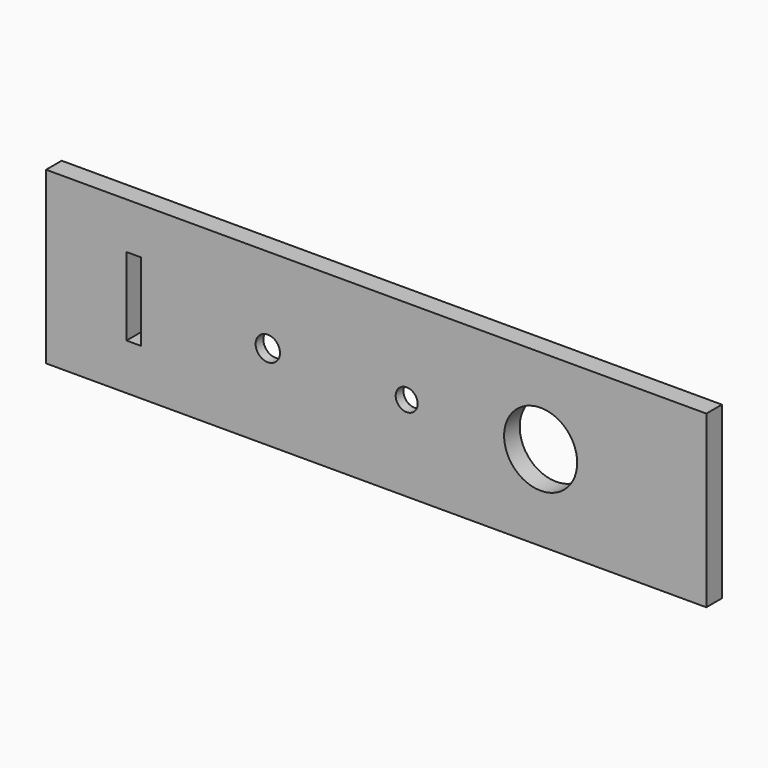
from build123d import *

# Parameters (mm, degrees)
F0_W          = 215.10625
F0_H          = 55.5625
F0_R          = 3.96875
F0_R_2        = 3.571875
F0_R_3        = 11.90625
F1_DEPTH      = 6.35
F2_W          = 4.7625
F2_H          = 25.4
F3_DEPTH      = 332
F3_DEPTH_BACK = 6.351
F5_DEPTH      = 3.175
F7_DEPTH      = 4.7625
F7_DEPTH_BACK = 3.175


# Not quite as in the source:
# - an extrude ends at something that could not be found from the text; its depth is read off the source's solid


with BuildPart() as f1:
    # F0 (on Front) → F1 (new body)
    with BuildSketch(Plane.XZ):
        with Locations((107.553125, 27.78125)):
            Rectangle(F0_W, F0_H)
        with Locations((72.23125, 27.7749)):
            Circle(F0_R, mode=Mode.SUBTRACT)
        with Locations((117.475, 27.78125)):
            Circle(F0_R_2, mode=Mode.SUBTRACT)
        with Locations((161.13125, 27.78125)):
            Circle(F0_R_3, mode=Mode.SUBTRACT)
    extrude(amount=F1_DEPTH)

    # F2 (on face) → F3 (cut, two sides)
    with BuildSketch(Plane.XZ.offset(6.35)) as f3_sk:
        with Locations((28.575, 27.78125)):
            Rectangle(F2_W, F2_H)
    extrude(amount=F3_DEPTH, mode=Mode.SUBTRACT)
    extrude(f3_sk.sketch, amount=-F3_DEPTH_BACK, mode=Mode.SUBTRACT)

    # F4 (on face) → F5 (cut)
    with BuildSketch(Plane.XZ):
        with BuildLine():
            Line((57.15, 10.3124), (130.175, 10.3124))
            ThreePointArc((130.175, 10.3124), (136.9101920908, 13.1022079092), (139.7, 19.8374))
            Line((139.7, 19.8374), (139.7, 35.7124))
            ThreePointArc((139.7, 35.7124), (136.9101920908, 42.4475920908), (130.175, 45.2374))
            Line((130.175, 45.2374), (57.15, 45.2374))
            ThreePointArc((57.15, 45.2374), (50.4148079092, 42.4475920908), (47.625, 35.7124))
            Line((47.625, 35.7124), (47.625, 19.8374))
            ThreePointArc((47.625, 19.8374), (50.4148079092, 13.1022079092), (57.15, 10.3124))
        make_face()
    extrude(amount=F5_DEPTH, mode=Mode.SUBTRACT)

    # F6 (on face) → F7 (cut, two sides)
    with BuildSketch(Plane.XZ) as f7_sk:
        with BuildLine():
            Line((69.05625, 15.0749), (75.40625, 15.0749))
            ThreePointArc((75.40625, 15.0749), (76.99375, 16.6624), (75.40625, 18.2499))
            Line((75.40625, 18.2499), (69.05625, 18.2499))
            ThreePointArc((69.05625, 18.2499), (67.46875, 16.6624), (69.05625, 15.0749))
        make_face()
    extrude(amount=F7_DEPTH, mode=Mode.SUBTRACT)
    extrude(f7_sk.sketch, amount=-F7_DEPTH_BACK, mode=Mode.SUBTRACT)


solid = f1.part
